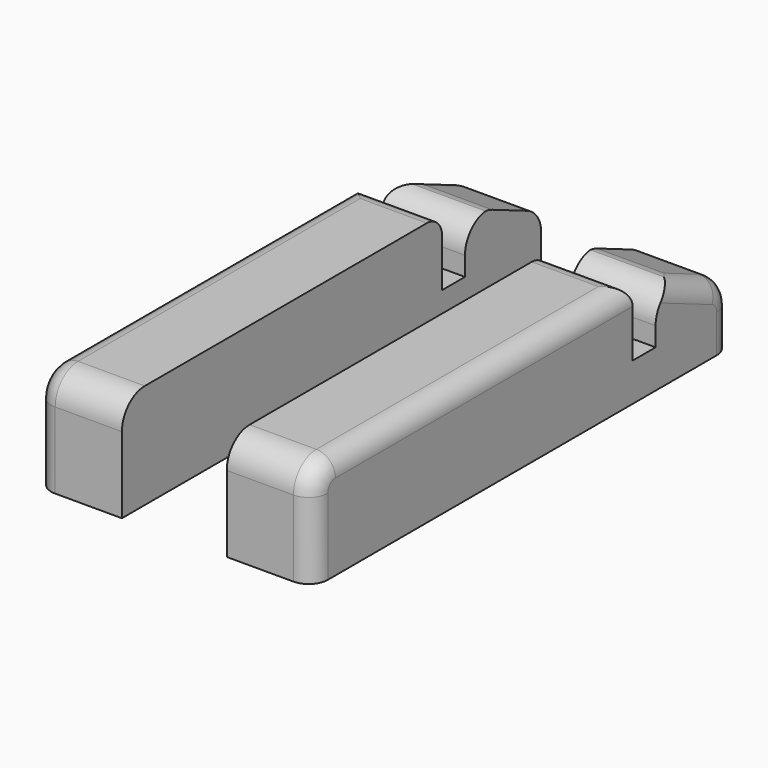
from build123d import *

# Parameters (mm, degrees)
F0_W         = 9
F0_H         = 3
F1_DEPTH     = 4
F0_H_2       = 10
F2_DEPTH     = 9
F0_H_3       = 42
F3_DEPTH     = 11
F4_SIZE2     = 3
F4_SIZE      = 7
F5_T1_DEPTH  = 24
F5_T3_DEPTH  = 18.8909423697
F5_T5_DEPTH  = 12.0788655293
F6_T1_DEPTH  = 19
F6_T3_DEPTH  = 44
F6_T5_DEPTH  = 10.021811526
F6_T7_DEPTH  = 13
F6_T9_DEPTH  = 9.0218115261
F6_T12_ANGLE = 90.0000000053
F6_T14_ANGLE = 66.8014094864


# Not quite as in the source:
# - a fillet or chamfer that OpenCascade refuses, or shapes differently, is made with other operations: its cross-section is extruded or revolved along the edge and cut away or added


with BuildPart() as f1:
    # F0 (on Top) → F1 (new body)
    with BuildSketch(Plane.XY):
        with Locations((0, 16)):
            Rectangle(F0_W, F0_H)
    extrude(amount=F1_DEPTH)

    # F0 (on Top) → F2 (join)
    with BuildSketch(Plane.XY):
        with Locations((0, 22.5)):
            Rectangle(F0_W, F0_H_2)
    extrude(amount=F2_DEPTH)

    # F0 (on Top) → F3 (join)
    with BuildSketch(Plane.XY):
        with Locations((0, -6.5)):
            Rectangle(F0_W, F0_H_3)
    extrude(amount=F3_DEPTH)

    # F4
    f4_edges = [f1.edges().sort_by_distance(p)[0] for p in [
        (0, 27.5, 9),
    ]]
    f4_side = f1.faces().sort_by_distance((0, 22.5, 9))[0]
    chamfer(f4_edges, length=F4_SIZE, length2=F4_SIZE2, reference=f4_side)

    # F5: fillet of radius 3 on 4 edges, made by hand

    # F5_s2 → F5_t1 (cut)
    with BuildSketch(Plane.YZ.offset(-12)):
        with BuildLine():
            ThreePointArc((20.5, 9), (18.3786796564, 8.1213203436), (17.5, 6))
            Line((17.5, 6), (17.5, 9))
            Line((17.5, 9), (20.5, 9))
        make_face()
        with BuildLine():
            ThreePointArc((-27.5, 8), (-26.6213203436, 10.1213203436), (-24.5, 11))
            Line((-24.5, 11), (-27.5, 11))
            Line((-27.5, 11), (-27.5, 8))
        make_face()
    extrude(amount=F5_T1_DEPTH, mode=Mode.SUBTRACT)

    # F5_s4 → F5_t3 (cut)
    with BuildSketch(Plane.YZ.offset(-9.4454711849)):
        with BuildLine():
            ThreePointArc((25.6817578957, 6.7792466161), (27.0045232767, 5.6732845523), (27.5, 4.0218115261))
            Line((27.5, 4.0218115261), (27.5, 6))
            Line((27.5, 6), (25.6817578957, 6.7792466161))
        make_face()
    extrude(amount=F5_T3_DEPTH, mode=Mode.SUBTRACT)

    # F5_s6 → F5_t5 (cut)
    with BuildSketch(Plane.YZ.offset(-6.0394327647)):
        with BuildLine():
            ThreePointArc((19.8842268941, 9), (20.4874245109, 8.9387331684), (21.0659847899, 8.7574350901))
            Line((21.0659847899, 8.7574350901), (20.5, 9))
            Line((20.5, 9), (19.8842268941, 9))
        make_face()
    extrude(amount=F5_T5_DEPTH, mode=Mode.SUBTRACT)

    # F6: fillet of radius 2 on 7 edges, made by hand

    # F6_s2 → F6_t1 (cut)
    with BuildSketch(Plane.YZ.offset(-9.5)):
        with BuildLine():
            ThreePointArc((14.5, 9), (13.9142135624, 10.4142135624), (12.5, 11))
            Line((12.5, 11), (14.5, 11))
            Line((14.5, 11), (14.5, 9))
        make_face()
    extrude(amount=F6_T1_DEPTH, mode=Mode.SUBTRACT)

    # F6_s4 → F6_t3 (cut)
    with BuildSketch(Plane.XZ.offset(-19.5)):
        with BuildLine():
            ThreePointArc((-2.5, 11), (-3.9142135624, 10.4142135624), (-4.5, 9))
            Line((-4.5, 9), (-4.5, 11))
            Line((-4.5, 11), (-2.5, 11))
        make_face()
    extrude(amount=F6_T3_DEPTH, mode=Mode.SUBTRACT)

    # F6_s6 → F6_t5 (cut)
    with BuildSketch(Plane(origin=(0, 10.0306044674, -4.298830486), x_dir=(1, 0, 0), z_dir=(0, 0.91914503, -0.3939192986))):
        with BuildLine():
            ThreePointArc((-2.5, -16.347650891), (-3.9142135624, -15.7618644534), (-4.5, -14.347650891))
            Line((-4.5, -14.347650891), (-4.5, -16.347650891))
            Line((-4.5, -16.347650891), (-2.5, -16.347650891))
        make_face()
    extrude(amount=F6_T5_DEPTH, mode=Mode.SUBTRACT)

    # F6_s8 → F6_t7 (cut)
    with BuildSketch(Plane.XY.offset(-5)):
        with BuildLine():
            ThreePointArc((-2.5, -27.5), (-3.9142135624, -26.9142135624), (-4.5, -25.5))
            Line((-4.5, -25.5), (-4.5, -27.5))
            Line((-4.5, -27.5), (-2.5, -27.5))
        make_face()
    extrude(amount=F6_T7_DEPTH, mode=Mode.SUBTRACT)

    # F6_s10 → F6_t9 (cut)
    with BuildSketch(Plane.XY.offset(-5)):
        with BuildLine():
            ThreePointArc((-2.5, 27.5), (-3.9142135624, 26.9142135624), (-4.5, 25.5))
            Line((-4.5, 25.5), (-4.5, 27.5))
            Line((-4.5, 27.5), (-2.5, 27.5))
        make_face()
    extrude(amount=F6_T9_DEPTH, mode=Mode.SUBTRACT)

    # F6_s11 → F6_t12 (revolve, cut)
    with BuildSketch(Plane.XY.offset(8.0000000001)):
        with BuildLine():
            ThreePointArc((-2.5, -27.5), (-3.9142135624, -26.9142135624), (-4.5, -25.5))
            Line((-4.5, -25.5), (-4.5, -27.5))
            Line((-4.5, -27.5), (-2.5, -27.5))
        make_face()
    revolve(axis=Axis((-4.5, -24.5000000001, 8.0000000001), (-1, 0, 0)), revolution_arc=F6_T12_ANGLE, mode=Mode.SUBTRACT)

    # F6_s13 → F6_t14 (revolve, cut)
    with BuildSketch(Plane(origin=(0, 19.2421027237, -8.2466154526), x_dir=(1, 0, 0), z_dir=(0, -0.91914503, 0.3939192986))):
        with BuildLine():
            ThreePointArc((-2.5, 16.3476508906), (-3.9142135624, 15.761864453), (-4.5, 14.3476508906))
            Line((-4.5, 14.3476508906), (-4.5, 16.3476508906))
            Line((-4.5, 16.3476508906), (-2.5, 16.3476508906))
        make_face()
    revolve(axis=Axis((-4.5, 24.5, 4.021811526), (-1, 0, 0)), revolution_arc=F6_T14_ANGLE, mode=Mode.SUBTRACT)


with BuildPart() as f8_1:
    # F8: instance of F1
    add(f1.part.mirror(Plane.YZ.offset(10)))


solid = Compound([f1.part, f8_1.part])
